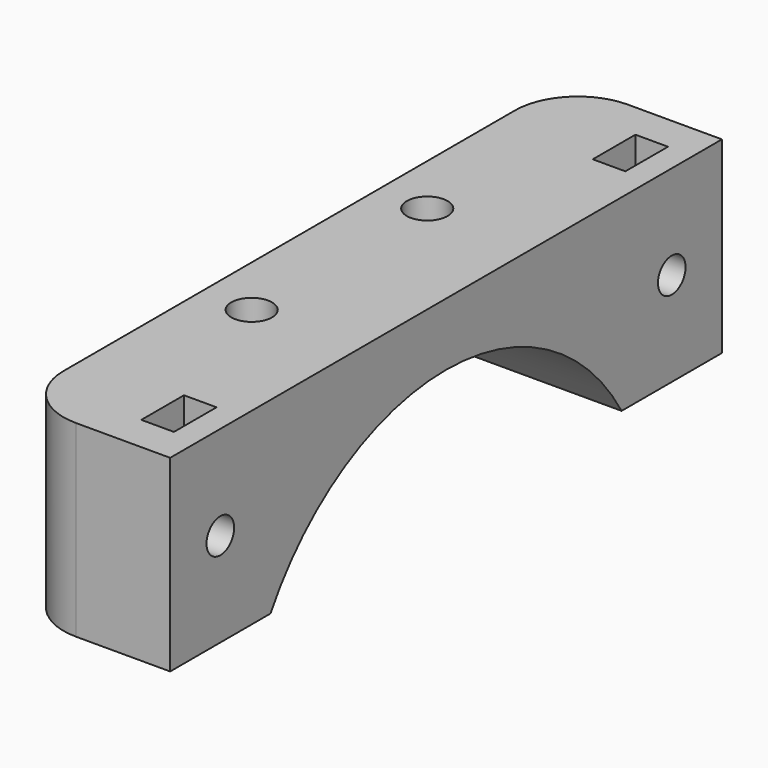
from build123d import *

# Parameters (mm, degrees)
F0_W           = 110
F0_H           = 30
F1_DEPTH       = 12.5
F3_D           = 5.5
F3_DEPTH       = 12
F3_TIP         = 1.6523667023
F5_DEPTH       = 25
F7_D           = 6.5
F10_DEPTH      = 3
F10_DEPTH_BACK = 20.0010001
F11_W          = 5.2
F11_H          = 8.5
F12_DEPTH      = 20
F13_R          = 10


# Not quite as in the source:
# - a pattern or mirror of a feature is missing from the dataset's text; its kind, count and spacing are read off the source's solid


with BuildPart() as f1:
    # F0 (on Right) → F1 (new body, symmetric)
    with BuildSketch(Plane.YZ):
        with Locations((0, 15)):
            Rectangle(F0_W, F0_H)
    extrude(amount=F1_DEPTH, both=True)

    # F3
    with Locations(Plane.YZ.offset(12.5)):
        with Locations((-45, 15), (45, 15)):
            Hole(F3_D / 2, depth=F3_DEPTH)
            with Locations((0, 0, -(F3_DEPTH + F3_TIP / 2))):  # 118° drill point
                Cone(0, F3_D / 2, F3_TIP, mode=Mode.SUBTRACT)

    # F4 (on face) → F5 (cut, through all)
    with BuildSketch(Plane.YZ.offset(12.5)):
        with BuildLine():
            Line((-35, 0), (35, 0))
            ThreePointArc((35, 0), (0, 20), (-35, 0))
        make_face()
    extrude(amount=-F5_DEPTH, mode=Mode.SUBTRACT)

    # F7 (through all)
    with Locations(Plane.XY.offset(30)):
        with Locations((-4.5, 17.5), (-4.5, -17.5)):
            Hole(F7_D / 2)

    # F9 (on offset) → F10 (cut, two sides)
    with BuildSketch(Plane.XY.offset(20)) as f10_sk:
        Polygon((-9.75, -20.5310889132), (-4.5, -23.5621778265), (0.75, -20.5310889132), (0.75, -14.4689110868), (-4.5, -11.4378221735), (-9.75, -14.4689110868), align=None)
    f10 = extrude(amount=F10_DEPTH, mode=Mode.SUBTRACT) + extrude(f10_sk.sketch, amount=-F10_DEPTH_BACK, mode=Mode.SUBTRACT)

    # F10_copies: F10 across plane
    add(f10.mirror(Plane.ZX), mode=Mode.SUBTRACT)

    # F11 (on face) → F12 (cut)
    with BuildSketch(Plane.XY.offset(30)):
        with Locations((5.9, -45)):
            Rectangle(F11_W, F11_H)
    f12 = extrude(amount=-F12_DEPTH, mode=Mode.SUBTRACT)

    # F12_copies: F12 across plane
    add(f12.mirror(Plane.ZX), mode=Mode.SUBTRACT)

    # F13
    f13_edges = [f1.edges().sort_by_distance(p)[0] for p in [
        (-12.5, -55, 15),
        (-12.5, 55, 15),
    ]]
    fillet(f13_edges, radius=F13_R)


solid = f1.part
